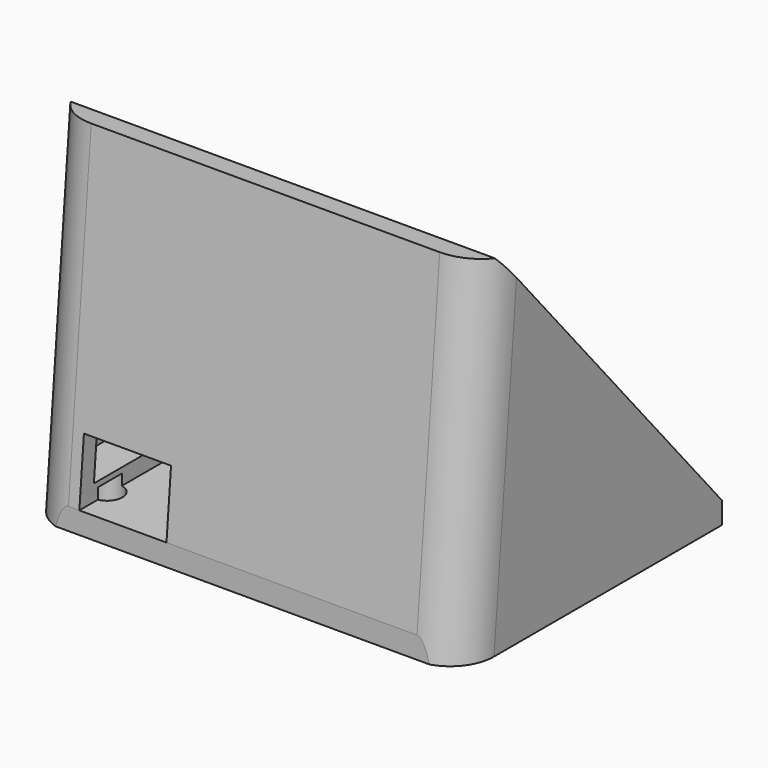
from build123d import *

# Parameters (mm, degrees)
F1_DEPTH     = 40
F2_T         = -1.5
F0_W         = 30
F0_H         = 2
F3_DEPTH     = 40
F4_W         = 8
F4_H         = 6
F5_DEPTH     = 10
F6_R         = 1.4
F7_DEPTH     = 3
F8_T4_DEPTH  = 36.8630372484
F8_T11_DEPTH = 36.8630372484
F8_T17_DEPTH = 36.8630372484
F8_T20_DEPTH = 90


# Not quite as in the source:
# - a fillet or chamfer that OpenCascade refuses, or shapes differently, is made with other operations: its cross-section is extruded or revolved along the edge and cut away or added


with BuildPart() as f1:
    # F0 (on Right) → F1 (new body)
    with BuildSketch(Plane.YZ):
        Polygon((2.6146722824, 29.8858409428), (0, 0), (30, 0), (4.6070616786, 29.7115294573), align=None)
    extrude(amount=F1_DEPTH)

    # F2
    f2_openings = [f1.faces().sort_by_distance(p)[0] for p in [
        (20, 17.303531, 14.855765),
    ]]
    offset(amount=F2_T, openings=f2_openings)

    # F0 (on Right) → F3 (join)
    with BuildSketch(Plane.YZ):
        with Locations((15, -1)):
            Rectangle(F0_W, F0_H)
    extrude(amount=F3_DEPTH)

    # F4 (on Front) → F5 (cut)
    with BuildSketch(Plane.XZ):
        with Locations((9, 3)):
            Rectangle(F4_W, F4_H)
    extrude(amount=-F5_DEPTH, mode=Mode.SUBTRACT)

    # F6 (on face) → F7 (cut)
    with BuildSketch(Plane(origin=(0, 0, -2), x_dir=(1, 0, 0), z_dir=(0, 0, -1))):
        with Locations((4.75, -3.5)):
            Circle(F6_R)
        with Locations((35.25, -3.5)):
            Circle(F6_R)
    extrude(amount=-F7_DEPTH, mode=Mode.SUBTRACT)

    # F8: fillet of radius 4 on 4 edges, made by hand


with BuildPart() as f8_tool2:
    # F8_s3 → F8_t4 (new body)
    with BuildSketch(Plane(origin=(0, -0.728886723, -8.3312133668), x_dir=(1, 0, 0), z_dir=(0, 0.0871557427, 0.9961946981))):
        with BuildLine():
            ThreePointArc((5.5, 1.5), (2.6715728753, 2.6715728753), (1.5, 5.5))
            Line((1.5, 5.5), (1.5, 1.5))
            Line((1.5, 1.5), (5.5, 1.5))
        make_face()
    extrude(amount=F8_T4_DEPTH)

    split(bisect_by=Plane.YZ.offset(5), keep=Keep.BOTTOM)

    split(bisect_by=Plane(origin=(0, 17.3367768884, 14.8168645055), x_dir=(1, 0, 0), z_dir=(0, -0.7601924513, -0.6496979583)), keep=Keep.TOP)

    split(bisect_by=Plane.XY.offset(1.5), keep=Keep.TOP)


with BuildPart() as f1_1:
    add(f1.part)

    # F8_t1: union F8_tool2
    add(f8_tool2.part)


with BuildPart() as f8_tool9:
    # F8_s10 → F8_t11 (new body)
    with BuildSketch(Plane(origin=(0, -0.728886723, -8.3312133668), x_dir=(1, 0, 0), z_dir=(0, 0.0871557427, 0.9961946981))):
        with BuildLine():
            ThreePointArc((5.5, 1.5), (2.6715728753, 2.6715728753), (1.5, 5.5))
            Line((1.5, 5.5), (1.5, 1.5))
            Line((1.5, 1.5), (5.5, 1.5))
        make_face()
    extrude(amount=F8_T11_DEPTH)

    split(bisect_by=Plane.XY.offset(6), keep=Keep.TOP)

    split(bisect_by=Plane(origin=(0, 17.3367768884, 14.8168645055), x_dir=(1, 0, 0), z_dir=(0, -0.7601924513, -0.6496979583)), keep=Keep.TOP)


with BuildPart() as f1_2:
    add(f1_1.part)

    # F8_t8: union F8_tool9
    add(f8_tool9.part)


with BuildPart() as f8_tool15:
    # F8_s16 → F8_t17 (new body)
    with BuildSketch(Plane(origin=(0, -0.728886723, -8.3312133668), x_dir=(1, 0, 0), z_dir=(0, 0.0871557427, 0.9961946981))):
        with BuildLine():
            ThreePointArc((34.5, 1.5), (37.3284271247, 2.6715728753), (38.5, 5.5))
            Line((38.5, 5.5), (38.5, 1.5))
            Line((38.5, 1.5), (34.5, 1.5))
        make_face()
    extrude(amount=F8_T17_DEPTH)

    split(bisect_by=Plane(origin=(0, 17.3367768884, 14.8168645055), x_dir=(1, 0, 0), z_dir=(0, -0.7601924513, -0.6496979583)), keep=Keep.TOP)

    split(bisect_by=Plane.XY.offset(1.5), keep=Keep.TOP)


with BuildPart() as f1_3:
    add(f1_2.part)

    # F8_t14: union F8_tool15
    add(f8_tool15.part)

    # F8_s21 → F8_t20 (cut)
    with BuildSketch(Plane(origin=(0, 3.4862297099, 39.8477879237), x_dir=(1, 0, 0), z_dir=(0, -0.0871557427, -0.9961946981))):
        with BuildLine():
            ThreePointArc((4, 0), (1.1715728753, -1.1715728753), (0, -4))
            Line((0, -4), (0, 0))
            Line((0, 0), (4, 0))
        make_face()
        with BuildLine():
            ThreePointArc((36, 0), (38.8284271247, -1.1715728753), (40, -4))
            Line((40, -4), (40, 0))
            Line((40, 0), (36, 0))
        make_face()
    extrude(amount=F8_T20_DEPTH, mode=Mode.SUBTRACT)


solid = f1_3.part
